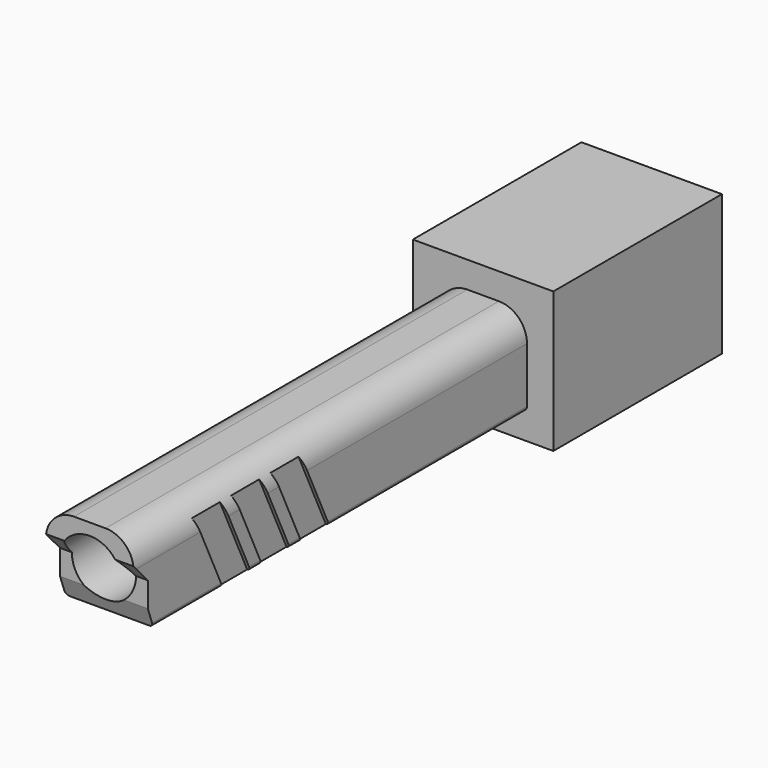
from build123d import *

# Parameters (mm, degrees)
F0_W        = 25.4
F0_H        = 25.4
F1_DEPTH    = 38.1
F0_R        = 5.8024107256
F2_DEPTH    = 127
F3_DEPTH    = 127
F5_DEPTH    = 0.635
F7_DEPTH    = 0.635
F8_F1_R     = 5.08
F8_F2_R     = 5.08
F9_T1_DEPTH = 29.2466340732
F9_T3_DEPTH = 49.2393659268
F9_T5_DEPTH = 11.684
F9_T7_DEPTH = 11.684
F11_DEPTH   = 25.4
F13_DEPTH   = 25.4


# Not quite as in the source:
# - a fillet or chamfer that OpenCascade refuses, or shapes differently, is made with other operations: its cross-section is extruded or revolved along the edge and cut away or added


with BuildPart() as f1:
    # F0 (on Front) → F1 (new body)
    with BuildSketch(Plane.XZ):
        Rectangle(F0_W, F0_H)
        Polygon((7.9375, 7.9375), (7.9375, 0), (7.9375, -7.9375), (0, -7.9375), (-7.9375, -7.9375), (-7.9375, 0), (-7.9375, 7.9375), (0, 7.9375), align=None, mode=Mode.SUBTRACT)
    extrude(amount=F1_DEPTH)



with BuildPart() as f1b:
    # F0 (on Front) → F1, piece 2 (new body)
    with BuildSketch(Plane.XZ):
        with BuildLine():
            ThreePointArc((0, -7.9375), (5.6126600757, -5.6126600757), (7.9375, 0))
            ThreePointArc((7.9375, 0), (5.6126600757, 5.6126600757), (0, 7.9375))
            ThreePointArc((0, 7.9375), (-5.6126600757, 5.6126600757), (-7.9375, 0))
            ThreePointArc((-7.9375, 0), (-5.6126600757, -5.6126600757), (0, -7.9375))
        make_face()
        Circle(F0_R, mode=Mode.SUBTRACT)
    extrude(amount=F1_DEPTH)


with BuildPart() as f1_1:
    add(f1.part)

    add(f1b.part)  # F2 merges F1b
    # F0 (on Front) → F2 (join)
    with BuildSketch(Plane.XZ):
        with BuildLine():
            ThreePointArc((0, -7.9375), (5.6126600757, -5.6126600757), (7.9375, 0))
            ThreePointArc((7.9375, 0), (5.6126600757, 5.6126600757), (0, 7.9375))
            ThreePointArc((0, 7.9375), (-5.6126600757, 5.6126600757), (-7.9375, 0))
            ThreePointArc((-7.9375, 0), (-5.6126600757, -5.6126600757), (0, -7.9375))
        make_face()
        Circle(F0_R, mode=Mode.SUBTRACT)
    extrude(amount=F2_DEPTH)

    # F0 (on Front) → F3 (join)
    with BuildSketch(Plane.XZ):
        with BuildLine():
            Line((7.9375, -7.9375), (7.9375, 0))
            ThreePointArc((7.9375, 0), (5.6126600757, -5.6126600757), (0, -7.9375))
            Line((0, -7.9375), (7.9375, -7.9375))
        make_face()
        with BuildLine():
            ThreePointArc((0, 7.9375), (5.6126600757, 5.6126600757), (7.9375, 0))
            Line((7.9375, 0), (7.9375, 7.9375))
            Line((7.9375, 7.9375), (0, 7.9375))
        make_face()
        with BuildLine():
            ThreePointArc((-7.9375, 0), (-5.6126600757, 5.6126600757), (0, 7.9375))
            Line((0, 7.9375), (-7.9375, 7.9375))
            Line((-7.9375, 7.9375), (-7.9375, 0))
        make_face()
        with BuildLine():
            Line((-7.9375, -7.9375), (0, -7.9375))
            ThreePointArc((0, -7.9375), (-5.6126600757, -5.6126600757), (-7.9375, 0))
            Line((-7.9375, 0), (-7.9375, -7.9375))
        make_face()
    extrude(amount=F3_DEPTH)

    # F4 (on face) → F5 (cut)
    with BuildSketch(Plane(origin=(-7.9375, 0, 0), x_dir=(0, -1, 0), z_dir=(-1, 0, 0))):
        Polygon((106.8973659268, -7.9375), (114.3, 7.9375), (107.95, 7.9375), (100.5473659268, -7.9375), align=None)
        Polygon((98.0073659268, -7.9375002533), (105.41, 7.9374997467), (99.06, 7.9374997467), (91.6573659268, -7.9375002533), align=None)
        Polygon((89.1173659268, -7.9375002533), (96.52, 7.9374997467), (90.17, 7.9374997467), (82.7673659268, -7.9375002533), align=None)
    extrude(amount=-F5_DEPTH, mode=Mode.SUBTRACT)

    # F6 (on face) → F7 (cut)
    with BuildSketch(Plane.YZ.offset(7.9375)):
        Polygon((-107.95, 7.9375), (-114.3, 7.9375), (-106.8973659268, -7.9375), (-100.5473659268, -7.9375), align=None)
        Polygon((-99.06, 7.9374997467), (-105.41, 7.9374997467), (-98.0073659268, -7.9375002533), (-91.6573659268, -7.9375002533), align=None)
        Polygon((-90.17, 7.9374997467), (-96.52, 7.9374997467), (-89.1173659268, -7.9375002533), (-82.7673659268, -7.9375002533), align=None)
    extrude(amount=-F7_DEPTH, mode=Mode.SUBTRACT)

    # F8: fillet of radius 5.08 on 8 edges, made by hand

    # F8_f1
    f8_f1_edges = [f1_1.edges().sort_by_distance(p)[0] for p in [
        (-7.9375, -120.65, 7.9375),
    ]]
    fillet(f8_f1_edges, radius=F8_F1_R)

    # F8_f2
    f8_f2_edges = [f1_1.edges().sort_by_distance(p)[0] for p in [
        (7.9375, -120.65, 7.9375),
    ]]
    fillet(f8_f2_edges, radius=F8_F2_R)

    # F9: fillet of radius 0.762 on 8 edges, made by hand

    # F9_s2 → F9_t1 (cut)
    with BuildSketch(Plane.XZ.offset(102.3253659268)):
        with BuildLine():
            ThreePointArc((-7.9375, -7.1755), (-7.7143153673, -7.7143153673), (-7.1755, -7.9375))
            Line((-7.1755, -7.9375), (-7.1755, -7.95274))
            Line((-7.1755, -7.95274), (-7.95274, -7.95274))
            Line((-7.95274, -7.95274), (-7.95274, -7.1755))
            Line((-7.95274, -7.1755), (-7.9375, -7.1755))
        make_face()
        with BuildLine():
            ThreePointArc((7.9375, -7.1755), (7.7143153673, -7.7143153673), (7.1755, -7.9375))
            Line((7.1755, -7.9375), (7.1755, -7.95274))
            Line((7.1755, -7.95274), (7.95274, -7.95274))
            Line((7.95274, -7.95274), (7.95274, -7.1755))
            Line((7.95274, -7.1755), (7.9375, -7.1755))
        make_face()
    extrude(amount=F9_T1_DEPTH, mode=Mode.SUBTRACT)

    # F9_s4 → F9_t3 (cut)
    with BuildSketch(Plane.XZ.offset(38.1)):
        with BuildLine():
            ThreePointArc((7.1755, -7.9375), (7.7143153673, -7.7143153673), (7.9375, -7.1755))
            Line((7.9375, -7.1755), (7.95274, -7.1755))
            Line((7.95274, -7.1755), (7.95274, -7.95274))
            Line((7.95274, -7.95274), (7.1755, -7.95274))
            Line((7.1755, -7.95274), (7.1755, -7.9375))
        make_face()
        with BuildLine():
            ThreePointArc((-7.1755, -7.9375), (-7.7143153673, -7.7143153673), (-7.9375, -7.1755))
            Line((-7.9375, -7.1755), (-7.95274, -7.1755))
            Line((-7.95274, -7.1755), (-7.95274, -7.95274))
            Line((-7.95274, -7.95274), (-7.1755, -7.95274))
            Line((-7.1755, -7.95274), (-7.1755, -7.9375))
        make_face()
    extrude(amount=F9_T3_DEPTH, mode=Mode.SUBTRACT)

    # F9_s6 → F9_t5 (cut)
    with BuildSketch(Plane.XZ.offset(84.5453659268)):
        with BuildLine():
            ThreePointArc((7.1755, -7.9375), (7.7143153673, -7.7143153673), (7.9375, -7.1755))
            Line((7.9375, -7.1755), (7.95274, -7.1755))
            Line((7.95274, -7.1755), (7.95274, -7.95274))
            Line((7.95274, -7.95274), (7.1755, -7.95274))
            Line((7.1755, -7.95274), (7.1755, -7.9375))
        make_face()
        with BuildLine():
            ThreePointArc((-7.1755, -7.9375), (-7.7143153673, -7.7143153673), (-7.9375, -7.1755))
            Line((-7.9375, -7.1755), (-7.95274, -7.1755))
            Line((-7.95274, -7.1755), (-7.95274, -7.95274))
            Line((-7.95274, -7.95274), (-7.1755, -7.95274))
            Line((-7.1755, -7.95274), (-7.1755, -7.9375))
        make_face()
    extrude(amount=F9_T5_DEPTH, mode=Mode.SUBTRACT)

    # F9_s8 → F9_t7 (cut)
    with BuildSketch(Plane.XZ.offset(93.4353659268)):
        with BuildLine():
            ThreePointArc((7.1755, -7.9375), (7.7143153673, -7.7143153673), (7.9375, -7.1755))
            Line((7.9375, -7.1755), (7.95274, -7.1755))
            Line((7.95274, -7.1755), (7.95274, -7.95274))
            Line((7.95274, -7.95274), (7.1755, -7.95274))
            Line((7.1755, -7.95274), (7.1755, -7.9375))
        make_face()
        with BuildLine():
            ThreePointArc((-7.1755, -7.9375), (-7.7143153673, -7.7143153673), (-7.9375, -7.1755))
            Line((-7.9375, -7.1755), (-7.95274, -7.1755))
            Line((-7.95274, -7.1755), (-7.95274, -7.95274))
            Line((-7.95274, -7.95274), (-7.1755, -7.95274))
            Line((-7.1755, -7.95274), (-7.1755, -7.9375))
        make_face()
    extrude(amount=F9_T7_DEPTH, mode=Mode.SUBTRACT)

    # F10 (on face) → F11 (cut)
    with BuildSketch(Plane(origin=(-7.9375, 0, 0), x_dir=(0, -1, 0), z_dir=(-1, 0, 0))):
        Polygon((139.3916606903, 2.8575), (129.1201191025, 15.1211110401), (129.6502673187, -9.5306912246), align=None)
    extrude(amount=-F11_DEPTH, mode=Mode.SUBTRACT)

    # F12 (on face) → F13 (cut)
    with BuildSketch(Plane(origin=(-7.9375, 0, 0), x_dir=(0, -1, 0), z_dir=(-1, 0, 0))):
        Polygon((131.4901411533, -9.1816671193), (131.4901411533, 8.4584709257), (123.7966120243, 0), (123.7966120243, -4.5106001198), (121.0489347577, -12.0942108333), align=None)
    extrude(amount=-F13_DEPTH, mode=Mode.SUBTRACT)


solid = f1_1.part
